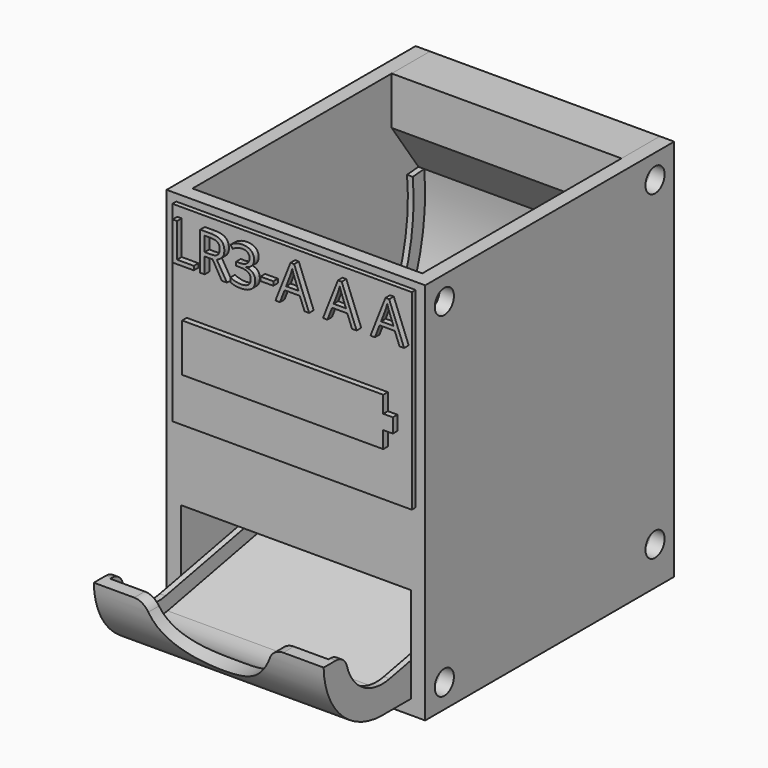
from build123d import *

# Parameters (mm, degrees)
F1_DEPTH     = 80
F2_W         = 48
F2_H         = 20
F3_DEPTH     = 65.001
F4_DEPTH     = 11.8
F5_W         = 50
F5_H         = 40
F6_DEPTH     = 1
F7_DEPTH     = 1
F10_DEPTH    = 1.2
F8_TEXT_SIZE = 11.1111111111
F11_DEPTH    = 1.2
F12_W        = 48
F12_H        = 3
F13_DEPTH    = 15
F15_DEPTH    = 24
F16_R        = 2.5
F17_DEPTH    = 30
F18_W        = 1.2
F18_H        = 3
F22_DEPTH    = 22.7580585408
F23_R        = 3.1
F24_R        = 3


# Not quite as in the source:
# - Text() gives the source's letters only with a copy of the font that has no kerning and outlines rounded to 1/6400 em; it was checked with that copy


with BuildPart() as f1:
    # F0 (on Top) → F1 (new body)
    with BuildSketch(Plane.XY):
        Polygon((-24, 65), (-27, 65), (-27, 0), (27, 0), (27, 65), (24, 65), (24, 3), (-24, 3), align=None)
    extrude(amount=F1_DEPTH)

    # F2 (on face) → F3 (cut, through all)
    with BuildSketch(Plane.XZ):
        with Locations((0, 13)):
            Rectangle(F2_W, F2_H)
    extrude(amount=-F3_DEPTH, mode=Mode.SUBTRACT)

    # F4 (add): a face of the model
    f4_faces = [f1.faces().sort_by_distance(p)[0] for p in [
        (0, 3, 1.5),
    ]]
    extrude(f4_faces, amount=F4_DEPTH)

    # F5 (on face) → F6 (cut)
    with BuildSketch(Plane.XZ):
        with Locations((0, 58.5)):
            Rectangle(F5_W, F5_H)
    extrude(amount=-F6_DEPTH, mode=Mode.SUBTRACT)

    # F12 (on face) → F13 (join)
    with BuildSketch(Plane(origin=(0, 65, 0), x_dir=(-1, 0, 0), z_dir=(0, 1, 0))):
        with Locations((0, 1.5)):
            Rectangle(F12_W, F12_H)
    extrude(amount=-F13_DEPTH)


with BuildPart() as f7:
    # F5 (on face) → F7 (new body)
    with BuildSketch(Plane.XZ):
        with Locations((0, 58.5)):
            Rectangle(F5_W, F5_H)
    extrude(amount=F7_DEPTH)

    # F9 (on face) → F10 (join)
    with BuildSketch(Plane.XZ.offset(1)):
        Polygon((20, 58.5), (-22, 58.5), (-22, 48.5), (20, 48.5), (20, 52), (22, 52), (22, 55), (20, 55), align=None)
    extrude(amount=F10_DEPTH)

    # F8 (on face) → F11 (join)
    with BuildSketch(Plane.XZ.offset(1)):
        with Locations((-25.0755208333, 68.5)):
            Text('LR3-A A A', F8_TEXT_SIZE, font='Open Sans', text_align=(TextAlign.LEFT, TextAlign.BOTTOM))
    extrude(amount=F11_DEPTH)


with BuildPart() as f15:
    # F14 (on Right) → F15 (new body, symmetric)
    with BuildSketch(Plane.YZ):
        with BuildLine():
            Line((65, 3), (65, 80))
            Line((65, 80), (55, 80))
            Line((55, 80), (55, 70))
            Line((55, 70), (62, 60))
            ThreePointArc((62, 60), (53.6346037836, 29.3936067514), (26.8580673021, 12.3716134604))
            Line((26.8580673021, 12.3716134604), (-5, 6))
            ThreePointArc((-5, 6), (-15.2959173043, 8.5051033696), (-20, 18))
            Line((-20, 18), (-22.7570585408, 18))
            ThreePointArc((-22.7570585408, 18), (-18.1721426428, 7.3757151264), (-7.46, 3))
            Line((-7.46, 3), (65, 3))
        make_face()
    extrude(amount=F15_DEPTH, both=True)


with BuildPart() as f17_tool:
    # F16 (on Right) → F17 (new body, symmetric)
    with BuildSketch(Plane.YZ):
        with Locations((60, 75)):
            Circle(F16_R)
        with Locations((60, 8)):
            Circle(F16_R)
        with Locations((5, 75)):
            Circle(F16_R)
        with Locations((5, 5)):
            Circle(F16_R)
    extrude(amount=F17_DEPTH, both=True)


with BuildPart() as f1_1:
    add(f1.part)

    # F17: cut by f17_tool
    add(f17_tool.part, mode=Mode.SUBTRACT)


with BuildPart() as f15_1:
    add(f15.part)

    # F17: cut by f17_tool
    add(f17_tool.part, mode=Mode.SUBTRACT)

    # F19: sweep along a path in F19_path
    with BuildLine(Plane(origin=(24, -5, 6), x_dir=(0, 0, -1), z_dir=(-1, 0, 0))) as f19_path:
        ThreePointArc((-12, 15), (-2.5051033696, 10.2959173043), (0, 0))
        Line((0, 0), (-6.3716134604, -31.8580673021))
        ThreePointArc((-6.3716134604, -31.8580673021), (-23.3936067514, -58.6346037836), (-54, -67))
    # F18 (on face) → F19 (sweep)
    with BuildSketch(Plane.XY.offset(18)):
        with Locations((23.4, -18.5)):
            Rectangle(F18_W, F18_H)
    sweep(path=f19_path.line)

    # F20: sweep along a path in F20_path
    with BuildLine(Plane(origin=(-24, -5, 6), x_dir=(0, 0, -1), z_dir=(-1, 0, 0))) as f20_path:
        ThreePointArc((-12, 15), (-2.5051033696, 10.2959173043), (0, 0))
        Line((0, 0), (-6.3716134604, -31.8580673021))
        ThreePointArc((-6.3716134604, -31.8580673021), (-23.3936067514, -58.6346037836), (-54, -67))
    # F18 (on face) → F20 (sweep)
    with BuildSketch(Plane.XY.offset(18)):
        with Locations((-23.4, -18.5)):
            Rectangle(F18_W, F18_H)
    sweep(path=f20_path.line)

    # F21 (on Front) → F22 (cut, through all)
    with BuildSketch(Plane.XZ):
        with BuildLine():
            Line((13.416407865, 18), (-13.416407865, 18))
            ThreePointArc((-13.416407865, 18), (0, 8), (13.416407865, 18))
        make_face()
    extrude(amount=F22_DEPTH, mode=Mode.SUBTRACT)

    # F23
    f23_edges = [f15_1.edges().sort_by_distance(p)[0] for p in [
        (13.416408, -21.378529, 18),
        (-13.416408, -21.378529, 18),
    ]]
    fillet(f23_edges, radius=F23_R)

    # F24
    f24_edges = [f15_1.edges().sort_by_distance(p)[0] for p in [
        (-23.4, -17, 18),
        (23.4, -17, 18),
    ]]
    fillet(f24_edges, radius=F24_R)


solid = Compound([f7.part, f1_1.part, f15_1.part])
